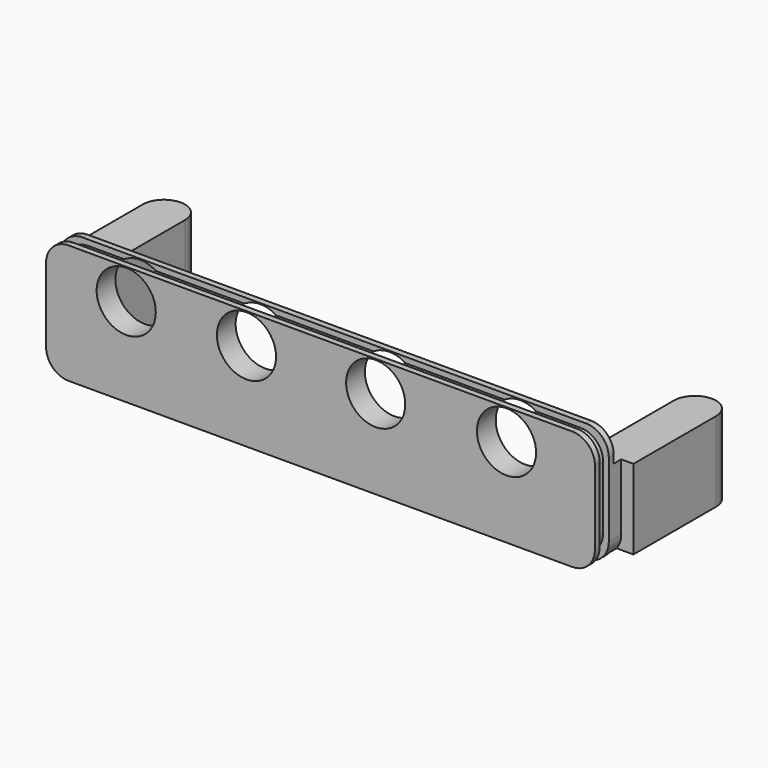
from build123d import *

# Parameters (mm, degrees)
F0_W      = 58.45
F0_H      = 12.7
F1_DEPTH  = 2.5
F2_W      = 58.45
F2_H      = 1.21
F6_DEPTH  = 0.6
F4_W      = 58.45
F4_H      = 1.21
F7_DEPTH  = 0.6
F5_W      = 1.21
F5_H      = 12.7
F8_DEPTH  = 0.6
F3_W      = 1.21
F3_H      = 12.7
F9_DEPTH  = 0.6
F10_W     = 3.2
F10_H     = 8.5
F11_DEPTH = 1
F12_R     = 2.4
F14_W     = 4.5
F14_H     = 8.5
F13_W     = 4.5
F13_H     = 8.5
F15_DEPTH = 13.25
F16_R     = 2.24999
F17_R     = 3.15
F18_DEPTH = 16.751


# Not quite as in the source:
# - a fillet or chamfer is up to 0.001 mm smaller than in the source, because OpenCascade refuses the exact size


with BuildPart() as f1:
    # F0 (on Front) → F1 (new body)
    with BuildSketch(Plane.XZ):
        Rectangle(F0_W, F0_H)
    extrude(amount=-F1_DEPTH)

    # F2 (on face) → F6 (cut)
    with BuildSketch(Plane.XY.offset(6.35)):
        with Locations((0, 1.245)):
            Rectangle(F2_W, F2_H)
    extrude(amount=-F6_DEPTH, mode=Mode.SUBTRACT)

    # F4 (on face) → F7 (cut)
    with BuildSketch(Plane(origin=(0, 0, -6.35), x_dir=(1, 0, 0), z_dir=(0, 0, -1))):
        with Locations((0, -1.245)):
            Rectangle(F4_W, F4_H)
    extrude(amount=-F7_DEPTH, mode=Mode.SUBTRACT)

    # F5 (on face) → F8 (cut)
    with BuildSketch(Plane.YZ.offset(29.225)):
        with Locations((1.245, 0)):
            Rectangle(F5_W, F5_H)
    extrude(amount=-F8_DEPTH, mode=Mode.SUBTRACT)

    # F3 (on face) → F9 (cut)
    with BuildSketch(Plane(origin=(-29.225, 0, 0), x_dir=(0, -1, 0), z_dir=(-1, 0, 0))):
        with Locations((-1.245, 0)):
            Rectangle(F3_W, F3_H)
    extrude(amount=-F9_DEPTH, mode=Mode.SUBTRACT)

    # F10 (on face) → F11 (join)
    with BuildSketch(Plane(origin=(0, 2.5, 0), x_dir=(-1, 0, 0), z_dir=(0, 1, 0))):
        with Locations((-27.625, -1.15)):
            Rectangle(F10_W, F10_H)
        with Locations((27.625, -1.15)):
            Rectangle(F10_W, F10_H)
    extrude(amount=F11_DEPTH)

    # F12
    f12_edges = [f1.edges().sort_by_distance(p)[0] for p in [
        (-29.225, 2.175, -6.35),
        (-28.625, 1.245, -5.75),
        (-29.225, 0.32, -6.35),
        (-29.225, 0.32, 6.35),
        (-28.625, 1.245, 5.75),
        (-29.225, 2.175, 6.35),
        (29.225, 0.32, 6.35),
        (28.625, 1.245, 5.75),
        (29.225, 2.175, 6.35),
        (29.225, 0.32, -6.35),
        (28.625, 1.245, -5.75),
        (29.225, 2.175, -6.35),
    ]]
    fillet(f12_edges, radius=F12_R)

    # F14 (on face) + F13 (on face) → F15 (join)
    with BuildSketch(Plane(origin=(0, 3.5, 0), x_dir=(-1, 0, 0), z_dir=(0, 1, 0))):
        with Locations((28.275, -1.15)):
            Rectangle(F14_W, F14_H)
    with BuildSketch(Plane(origin=(0, 3.5, 0), x_dir=(-1, 0, 0), z_dir=(0, 1, 0))):
        with Locations((-28.275, -1.15)):
            Rectangle(F13_W, F13_H)
    extrude(amount=F15_DEPTH)

    # F16 (radius 2.25 in the source; OpenCascade refuses exactly that, so slightly less here)
    f16_edges = [f1.edges().sort_by_distance(p)[0] for p in [
        (26.025, 16.75, -1.15),
        (30.525, 16.75, -1.15),
        (-26.025, 16.75, -1.15),
        (-30.525, 16.75, -1.15),
    ]]
    fillet(f16_edges, radius=F16_R)

    # F17 (on face) → F18 (cut, through all)
    with BuildSketch(Plane.XZ):
        with Locations((19.8096737738, 3.1)):
            Circle(F17_R)
        with Locations((5.8772991731, 3.1)):
            Circle(F17_R)
        with Locations((-7.8854865344, 3.1)):
            Circle(F17_R)
        with Locations((-20.6904198083, 3.1)):
            Circle(F17_R)
    extrude(amount=-F18_DEPTH, mode=Mode.SUBTRACT)


solid = f1.part
